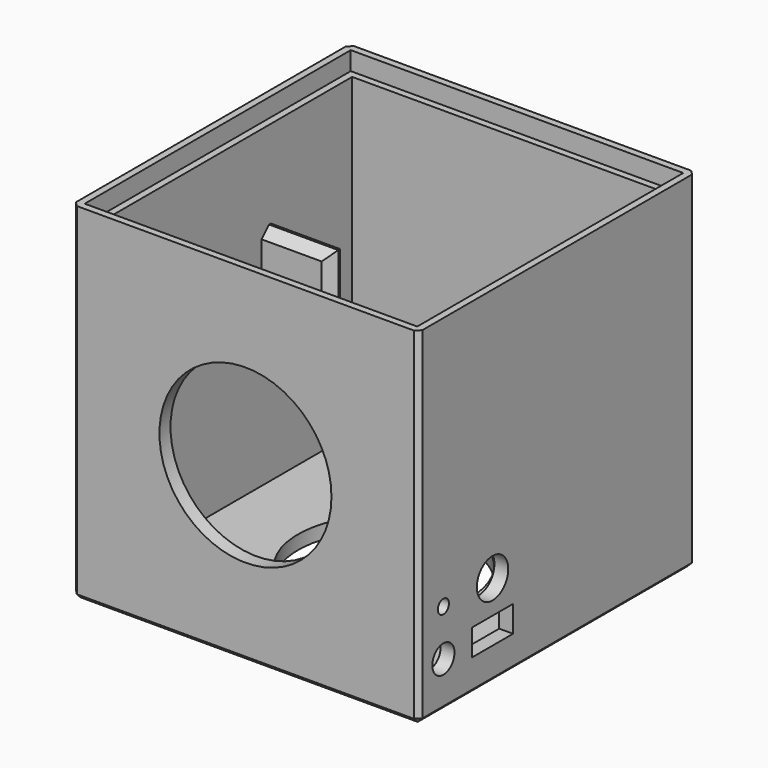
from build123d import *

# Parameters (mm, degrees)
F0_W           = 75
F0_H           = 75
F0_R           = 18.625
F1_DEPTH       = 3
F2_DEPTH       = 75
F3_R           = 18.625
F4_DEPTH       = 10.2
F0_W_2         = 15
F0_H_2         = 2.5
F5_DEPTH       = 77
F6_W           = 72
F6_H           = 72
F7_DEPTH       = 4
F8_SIZE        = 1
F10_W          = 12.5
F10_H          = 25
F11_DEPTH      = 25
F9_W           = 15
F9_H           = 25
F12_DEPTH      = 14.8
F14_DEPTH      = 3.8
F15_R          = 1.5
F15_R_2        = 4.25
F15_W          = 11.1
F15_H          = 5.7
F15_R_3        = 3
F16_DEPTH      = 25
F16_DEPTH_BACK = 25
F17_SIZE2      = 2
F17_SIZE       = 2


# Not quite as in the source:
# - a feature names something its author has since deleted; it is built from what else it names


with BuildPart() as f1:
    # F0 (on Top) → F1 (new body)
    with BuildSketch(Plane.XY):
        Rectangle(F0_W, F0_H)
        Polygon((-34.5, 12.5), (-34.5, 34.5), (29, 34.5), (31.5, 34.5), (34.5, 34.5), (34.5, -34.5), (-34.5, -34.5), (-34.5, 10), align=None, mode=Mode.SUBTRACT)
        Polygon((29, 34.5), (-34.5, 34.5), (-34.5, 12.5), (-19.5, 12.5), (-19.5, 10), (-34.5, 10), (-34.5, -34.5), (34.5, -34.5), (34.5, 34.5), (31.5, 34.5), (31.5, 10), (16.5, 10), (16.5, 12.5), (29, 12.5), align=None)
        Circle(F0_R, mode=Mode.SUBTRACT)
    extrude(amount=F1_DEPTH)

    # F0 (on Top) → F2 (join)
    with BuildSketch(Plane.XY):
        Rectangle(F0_W, F0_H)
        Polygon((-34.5, 12.5), (-34.5, 34.5), (29, 34.5), (31.5, 34.5), (34.5, 34.5), (34.5, -34.5), (-34.5, -34.5), (-34.5, 10), align=None, mode=Mode.SUBTRACT)
    extrude(amount=F2_DEPTH)

    # F3 (on face) → F4 (cut)
    with BuildSketch(Plane.XZ.offset(37.5)):
        with Locations((0, 37.5)):
            Circle(F3_R)
    extrude(amount=-F4_DEPTH, mode=Mode.SUBTRACT)

    # F0 (on Top) → F5 (join)
    with BuildSketch(Plane.XY):
        with Locations((-27, 11.25)):
            Rectangle(F0_W_2, F0_H_2)
        Polygon((31.5, 34.5), (29, 34.5), (29, 12.5), (16.5, 12.5), (16.5, 10), (31.5, 10), align=None)
    extrude(amount=F5_DEPTH)

    # F6 (on face) → F7 (cut)
    with BuildSketch(Plane.XY.offset(75)):
        Rectangle(F6_W, F6_H)
        Polygon((-34.5, 10), (-34.5, 12.5), (-34.5, 34.5), (29, 34.5), (31.5, 34.5), (34.5, 34.5), (34.5, -34.5), (-34.5, -34.5), align=None, mode=Mode.SUBTRACT)
    extrude(amount=-F7_DEPTH, mode=Mode.SUBTRACT)

    # F8
    f8_edges = [f1.edges().sort_by_distance(p)[0] for p in [
        (37.5, 0, 0),
        (0, -37.5, 0),
        (-37.5, -37.5, 37.5),
        (37.5, -37.5, 37.5),
        (-37.5, 0, 0),
        (0, 37.5, 0),
        (37.5, 37.5, 37.5),
        (-37.5, 37.5, 37.5),
    ]]
    chamfer(f8_edges, length=F8_SIZE)

    # F10 (on face) → F11 (cut)
    with BuildSketch(Plane(origin=(0, 12.5, 0), x_dir=(-1, 0, 0), z_dir=(0, 1, 0))):
        with Locations((-22.75, 64.5)):
            Rectangle(F10_W, F10_H)
        with Locations((-22.75, 15.5)):
            Rectangle(F10_W, F10_H)
    extrude(amount=-F11_DEPTH, mode=Mode.SUBTRACT)

    # F9 (on face) → F12 (cut)
    with BuildSketch(Plane.XZ.offset(-10)):
        Polygon((-19.5, 77), (-34.5, 77), (-34.5, 71), (-34.5, 52), (-19.5, 52), align=None)
        with Locations((-27, 15.5)):
            Rectangle(F9_W, F9_H)
    extrude(amount=-F12_DEPTH, mode=Mode.SUBTRACT)

    # F13 (on face) → F14 (cut)
    with BuildSketch(Plane(origin=(29, 0, 0), x_dir=(0, -1, 0), z_dir=(-1, 0, 0))):
        Polygon((-12.5, 52), (-10, 52), (-10, 77), (-34.5, 77), (-34.5, 71), (-34.5, 52), align=None)
        Polygon((-10, 28), (-12.5, 28), (-34.5, 28), (-34.5, 3), (-10, 3), align=None)
    extrude(amount=-F14_DEPTH, mode=Mode.SUBTRACT)

    # F15 (on face) → F16 (cut, two sides)
    with BuildSketch(Plane.YZ.offset(37.5)) as f16_sk:
        with Locations((-30.8012962341, 20)):
            Circle(F15_R)
        with Locations((-17.5, 20)):
            Circle(F15_R_2)
        with Locations((-17.5, 10)):
            Rectangle(F15_W, F15_H)
        with Locations((-30.8012962341, 10)):
            Circle(F15_R_3)
    extrude(amount=-F16_DEPTH, mode=Mode.SUBTRACT)
    extrude(f16_sk.sketch, amount=F16_DEPTH_BACK, mode=Mode.SUBTRACT)

    # F17
    f17_edges = [f1.edges().sort_by_distance(p)[0] for p in [
        (16.5, 10, 40),
        (24, 10, 52),
        (-27, 10, 52),
        (-19.5, 10, 40),
        (31.5, 22.25, 52),
    ]]
    chamfer(f17_edges, length=F17_SIZE, length2=F17_SIZE2)


solid = f1.part
